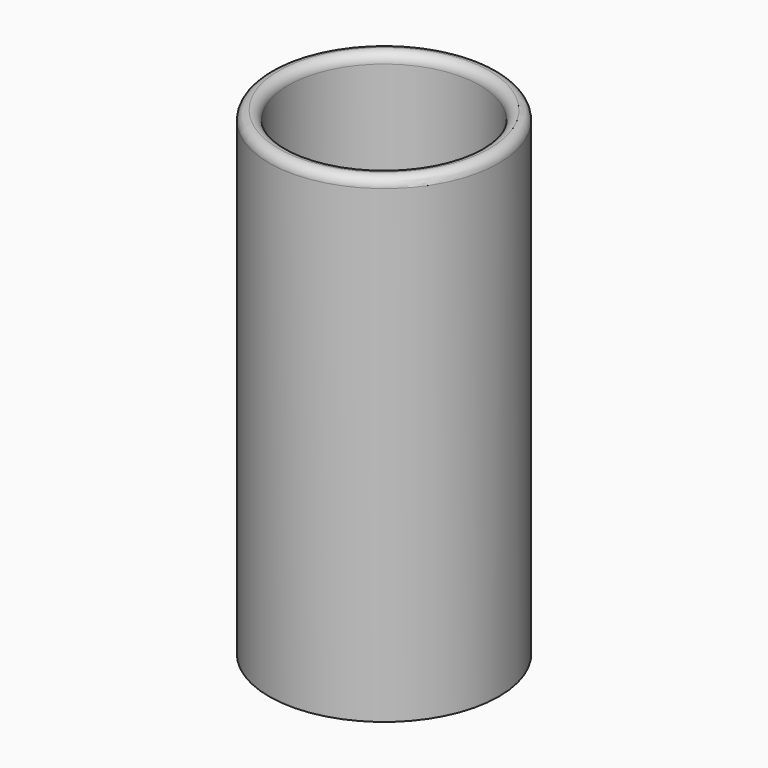
from build123d import *

# Parameters (mm, degrees)
F0_R     = 38.1
F1_DEPTH = 6.35
F2_R     = 38.1
F2_R_2   = 31.75
F3_DEPTH = 152.4
F4_R     = 3.17499


# Not quite as in the source:
# - a fillet or chamfer is up to 0.001 mm smaller than in the source, because OpenCascade refuses the exact size


with BuildPart() as f1:
    # F0 (on Top) → F1 (new body)
    with BuildSketch(Plane.XY):
        with Locations((-62.3559355736, 26.823958382)):
            Circle(F0_R)
    extrude(amount=F1_DEPTH)

    # F2 (on face) → F3 (join)
    with BuildSketch(Plane.XY.offset(6.35)):
        with Locations((-62.3559355736, 26.823958382)):
            Circle(F2_R)
        with Locations((-62.3559355736, 26.823958382)):
            Circle(F2_R_2, mode=Mode.SUBTRACT)
    extrude(amount=F3_DEPTH)

    # F4 (radius 3.175 in the source; OpenCascade refuses exactly that, so slightly less here)
    f4_edges = [f1.edges().sort_by_distance(p)[0] for p in [
        (-94.105936, 26.823958, 158.75),
        (-100.455936, 26.823958, 158.75),
    ]]
    fillet(f4_edges, radius=F4_R)


solid = f1.part
